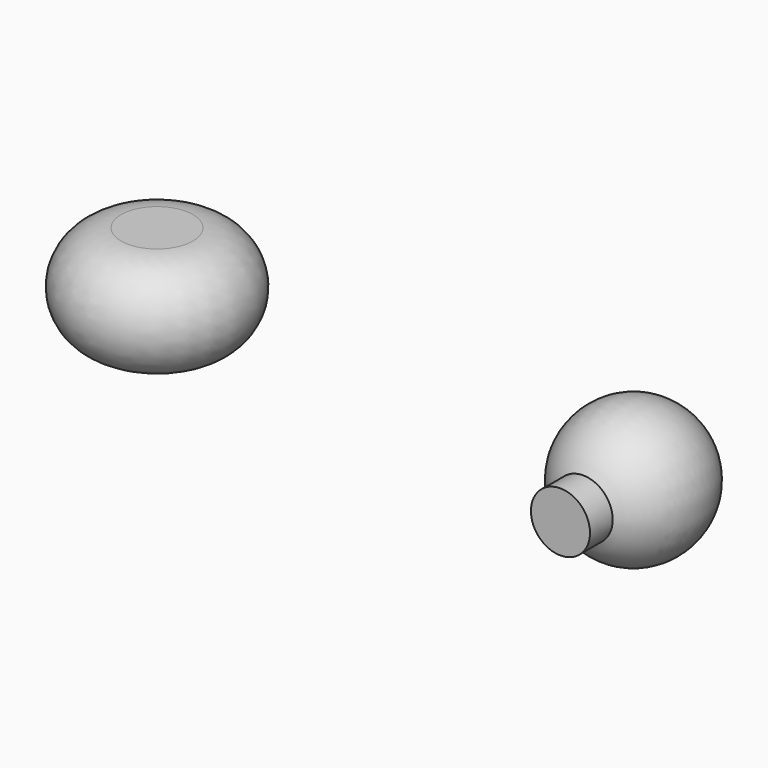
from build123d import *


with BuildPart() as f1:
    # F0 (on Top) → F1 (revolve)
    with BuildSketch(Plane.XY):
        with BuildLine():
            Line((33.8503696611, 74.7509705864), (33.7766118183, 34.5600933861))
            ThreePointArc((33.7766118183, 34.5600933861), (38.1658456195, 35.0501752748), (42.3420210759, 36.4872250916))
            ThreePointArc((42.3420210759, 36.4872250916), (53.3730726432, 59.0094067292), (33.8503696611, 74.7509705864))
        make_face()
        with BuildLine():
            Line((33.7766118183, 34.5600933861), (33.7650565687, 28.2636020438))
            Line((33.7650565687, 28.2636020438), (42.3420210759, 28.2636020438))
            Line((42.3420210759, 28.2636020438), (42.3420210759, 36.4872250916))
            ThreePointArc((42.3420210759, 36.4872250916), (38.1658456195, 35.0501752748), (33.7766118183, 34.5600933861))
        make_face()
    revolve(axis=Axis((33.8077131149, 51.5072863151, 0), (-0.0018351856, -0.999998316, 0)))


with BuildPart() as f3:
    # F2 (on Front) → F3 (revolve)
    with BuildSketch(Plane.XZ):
        with BuildLine():
            Line((-50.1620657742, 55.8738453063), (-60.5684927255, 55.8738453063))
            Line((-60.5684927255, 55.8738453063), (-60.5684927255, 25.8738453063))
            Line((-60.5684927255, 25.8738453063), (-50.5684927255, 25.8738453063))
            ThreePointArc((-50.5684927255, 25.8738453063), (-35.3652792498, 40.6706318307), (-50.1620657742, 55.8738453063))
        make_face()
    revolve(axis=Axis((-60.5684927255, 0, 40.8738453063), (0, 0, -1)))


solid = Compound([f1.part, f3.part])
